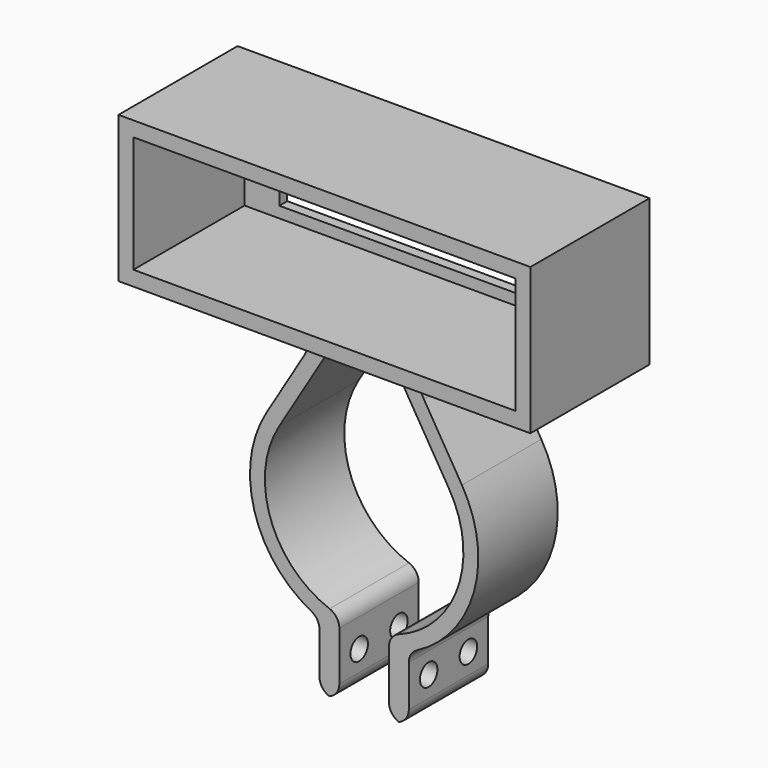
from build123d import *

# Parameters (mm, degrees)
F1_DEPTH    = 20
F3_DEPTH    = 20.001
F5_DEPTH    = 20
F6_T1_DEPTH = 20
F6_T3_DEPTH = 30.9947096091
F6_T5_DEPTH = 35
F7_W        = 83
F7_H        = 29.5
F7_W_2      = 77
F7_H_2      = 23.5
F8_DEPTH    = 30
F9_T1_DEPTH = 20
F10_R       = 2.2
F11_DEPTH   = 50.501
F12_W       = 77
F12_H       = 23.5
F12_W_2     = 63
F12_H_2     = 19
F13_DEPTH   = 2


# Not quite as in the source:
# - a fillet or chamfer that OpenCascade refuses, or shapes differently, is made with other operations: its cross-section is extruded or revolved along the edge and cut away or added


with BuildPart() as f1:
    # F0 (on Front) → F1 (new body)
    with BuildSketch(Plane.XZ):
        with BuildLine():
            ThreePointArc((8.5666506378, 30.3587301587), (0, 35.2), (-8.5666506378, 30.3587301587))
            Line((-8.5666506378, 30.3587301587), (-19.7032964668, 11.8650793651))
            ThreePointArc((-19.7032964668, 11.8650793651), (0, -23), (19.7032964668, 11.8650793651))
            Line((19.7032964668, 11.8650793651), (8.5666506378, 30.3587301587))
        make_face()
        with BuildLine():
            ThreePointArc((17.1333012755, 10.3174603175), (0, -20), (-17.1333012755, 10.3174603175))
            Line((-17.1333012755, 10.3174603175), (-5.9966554464, 28.8111111111))
            ThreePointArc((-5.9966554464, 28.8111111111), (0, 32.2), (5.9966554464, 28.8111111111))
            Line((5.9966554464, 28.8111111111), (17.1333012755, 10.3174603175))
        make_face(mode=Mode.SUBTRACT)
    extrude(amount=F1_DEPTH)

    # F2 (on face) → F3 (cut, through all)
    with BuildSketch(Plane.XZ.offset(20)):
        with BuildLine():
            ThreePointArc((5, -19.364916731), (0, -20), (-5, -19.364916731))
            Line((-5, -19.364916731), (-5, -22.4499443206))
            ThreePointArc((-5, -22.4499443206), (0, -23), (5, -22.4499443206))
            Line((5, -22.4499443206), (5, -19.364916731))
        make_face()
    extrude(amount=-F3_DEPTH, mode=Mode.SUBTRACT)

    # F4 (on Front) → F5 (join, through all)
    with BuildSketch(Plane.XZ):
        Polygon((-5, -34.4499443206), (-5, -22.4499443206), (-9, -21.1660104885), (-9, -34.4499443206), align=None)
        Polygon((5, -34.4499443206), (9, -34.4499443206), (9, -21.1660104885), (5, -22.4499443206), align=None)
    extrude(amount=F5_DEPTH)

    # F6: fillet of radius 3 on 8 edges, made by hand

    # F6_s2 → F6_t1 (join)
    with BuildSketch(Plane.XZ):
        with BuildLine():
            ThreePointArc((-9, -23.0651251893), (-9.4354487572, -21.5085016244), (-10.6153846154, -20.4037645906))
            ThreePointArc((-10.6153846154, -20.4037645906), (-9.8150946559, -20.8005749174), (-9, -21.1660104885))
            Line((-9, -21.1660104885), (-9, -23.0651251893))
        make_face()
        with BuildLine():
            ThreePointArc((9, -23.0651251893), (9.4354487572, -21.5085016244), (10.6153846154, -20.4037645906))
            ThreePointArc((10.6153846154, -20.4037645906), (9.8150946559, -20.8005749174), (9, -21.1660104885))
            Line((9, -21.1660104885), (9, -23.0651251893))
        make_face()
    extrude(amount=F6_T1_DEPTH)

    # F6_s4 → F6_t3 (cut)
    with BuildSketch(Plane.XZ.offset(-5.4973548045)):
        with BuildLine():
            ThreePointArc((-5, -21.5638586528), (-5.5372337928, -19.8507379307), (-6.9565217391, -18.7511814373))
            ThreePointArc((-6.9565217391, -18.7511814373), (-5.9861315369, -19.0831399204), (-5, -19.364916731))
            Line((-5, -19.364916731), (-5, -21.5638586528))
        make_face()
        with BuildLine():
            ThreePointArc((5, -21.5638586528), (5.5372337928, -19.8507379307), (6.9565217391, -18.7511814373))
            ThreePointArc((6.9565217391, -18.7511814373), (5.9861315369, -19.0831399204), (5, -19.364916731))
            Line((5, -19.364916731), (5, -21.5638586528))
        make_face()
    extrude(amount=F6_T3_DEPTH, mode=Mode.SUBTRACT)

    # F6_s6 → F6_t5 (cut)
    with BuildSketch(Plane.XZ.offset(-7.5)):
        with BuildLine():
            ThreePointArc((-8, -34.4499443206), (-5.8786796564, -33.5712646642), (-5, -31.4499443206))
            Line((-5, -31.4499443206), (-5, -34.4499443206))
            Line((-5, -34.4499443206), (-8, -34.4499443206))
        make_face()
        with BuildLine():
            ThreePointArc((5, -31.4499443206), (5.8786796564, -33.5712646642), (8, -34.4499443206))
            Line((8, -34.4499443206), (5, -34.4499443206))
            Line((5, -34.4499443206), (5, -31.4499443206))
        make_face()
        with BuildLine():
            ThreePointArc((6, -34.4499443206), (8.1213203436, -33.5712646642), (9, -31.4499443206))
            Line((9, -31.4499443206), (9, -34.4499443206))
            Line((9, -34.4499443206), (6, -34.4499443206))
        make_face()
        with BuildLine():
            ThreePointArc((-9, -31.4499443206), (-8.1213203436, -33.5712646642), (-6, -34.4499443206))
            Line((-6, -34.4499443206), (-9, -34.4499443206))
            Line((-9, -34.4499443206), (-9, -31.4499443206))
        make_face()
    extrude(amount=F6_T5_DEPTH, mode=Mode.SUBTRACT)

    # F7 (on Front) → F8 (join)
    with BuildSketch(Plane.XZ):
        with Locations((0, 46.95)):
            Rectangle(F7_W, F7_H)
        with Locations((0, 46.95)):
            Rectangle(F7_W_2, F7_H_2, mode=Mode.SUBTRACT)
    extrude(amount=F8_DEPTH)

    # F9: fillet of radius 5 on 2 edges, made by hand

    # F9_s2 → F9_t1 (join)
    with BuildSketch(Plane.XZ):
        with BuildLine():
            ThreePointArc((-16.3053853354, 32.2), (-11.9524078833, 29.659997419), (-12.0220600165, 24.6206349206))
            Line((-12.0220600165, 24.6206349206), (-11.5937274846, 24.3626984127))
            ThreePointArc((-11.5937274846, 24.3626984127), (-8.1383181059, 30.1007936508), (-6.7843570071, 31.85))
            Line((-6.7843570071, 31.85), (-7.1414284285, 32.7))
            Line((-7.1414284285, 32.7), (-16.3053853354, 32.7))
            Line((-16.3053853354, 32.7), (-16.3053853354, 32.2))
        make_face()
        with BuildLine():
            ThreePointArc((16.3053853354, 32.2), (11.9524078833, 29.659997419), (12.0220600165, 24.6206349206))
            Line((12.0220600165, 24.6206349206), (11.5937274846, 24.3626984127))
            ThreePointArc((11.5937274846, 24.3626984127), (8.1383181059, 30.1007936508), (6.7843570071, 31.85))
            Line((6.7843570071, 31.85), (7.1414284285, 32.7))
            Line((7.1414284285, 32.7), (16.3053853354, 32.7))
            Line((16.3053853354, 32.7), (16.3053853354, 32.2))
        make_face()
    extrude(amount=F9_T1_DEPTH)

    # F10 (on face) → F11 (cut, through all)
    with BuildSketch(Plane(origin=(-9, 0, 0), x_dir=(0, -1, 0), z_dir=(-1, 0, 0))):
        with Locations((5, -27.257534755)):
            Circle(F10_R)
        with Locations((15, -27.257534755)):
            Circle(F10_R)
    extrude(amount=-F11_DEPTH, mode=Mode.SUBTRACT)

    # F12 (on Front) → F13 (join)
    with BuildSketch(Plane.XZ):
        with Locations((0, 46.95)):
            Rectangle(F12_W, F12_H)
        with Locations((0, 46.95)):
            Rectangle(F12_W_2, F12_H_2, mode=Mode.SUBTRACT)
    extrude(amount=F13_DEPTH)


solid = f1.part
